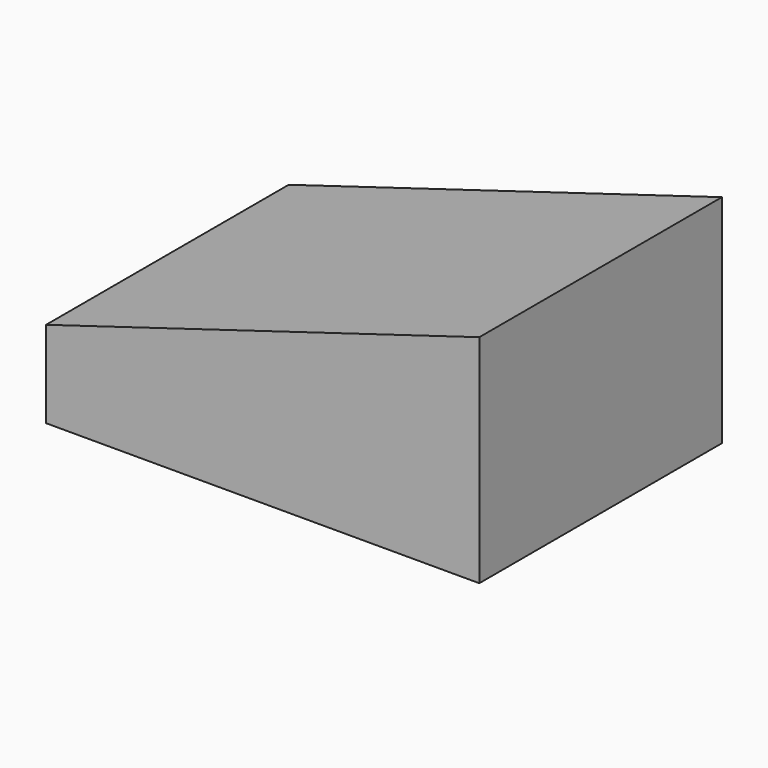
from build123d import *

# Parameters (mm, degrees)
F0_W     = 50
F0_H     = 25
F1_DEPTH = 35
F2_SIZE2 = 49.99999
F2_SIZE  = 14.99999


# Not quite as in the source:
# - a fillet or chamfer is up to 0.001 mm smaller than in the source, because OpenCascade refuses the exact size


with BuildPart() as f1:
    # F0 (on Front) → F1 (new body)
    with BuildSketch(Plane.XZ):
        with Locations((-25, 12.5)):
            Rectangle(F0_W, F0_H)
    extrude(amount=F1_DEPTH)

    # F2 (size 15 and 50 in the source; OpenCascade refuses exactly that, so slightly less here)
    f2_edges = [f1.edges().sort_by_distance(p)[0] for p in [
        (-50, -17.5, 25),
    ]]
    f2_side = f1.faces().sort_by_distance((-50, -17.5, 12.5))[0]
    chamfer(f2_edges, length=F2_SIZE, length2=F2_SIZE2, reference=f2_side)


solid = f1.part
